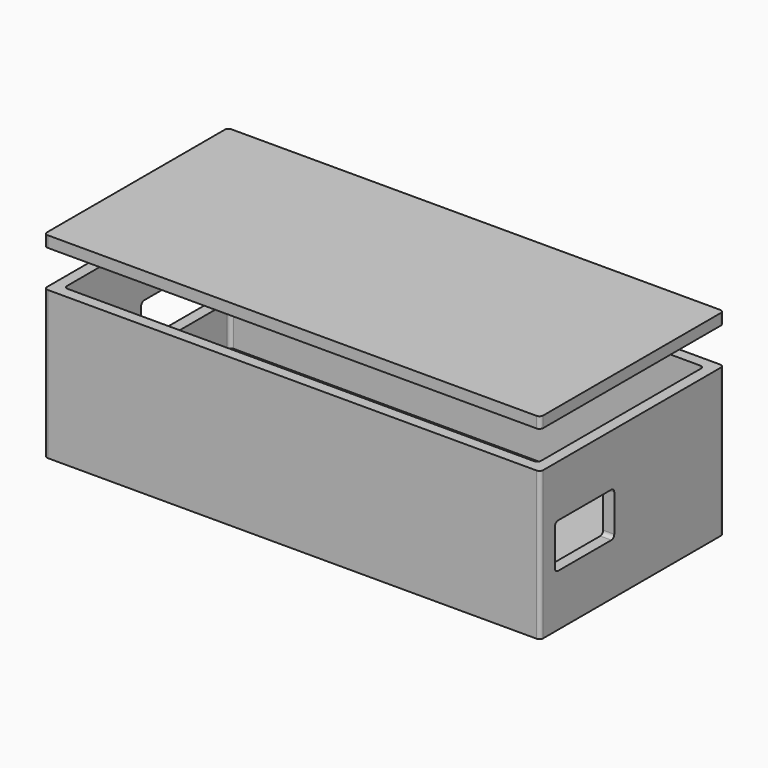
from build123d import *

# Parameters (mm, degrees)
F0_W      = 64
F0_H      = 28
F1_DEPTH  = 1.5
F0_W_2    = 67
F0_H_2    = 31
F2_DEPTH  = 20
F3_W      = 10
F3_H      = 6
F4_DEPTH  = 25
F5_W      = 14
F5_H      = 6
F6_DEPTH  = 25
F7_R      = 0.5
F8_R      = 0.5
F10_W     = 67
F10_H     = 31
F10_W_2   = 64
F10_H_2   = 28
F11_DEPTH = 1.5
F12_DEPTH = 1
F13_R     = 0.5


# Not quite as in the source:
# - a feature names something its author has since deleted; it is built from what else it names


with BuildPart() as f1:
    # F0 (on Top) → F1 (new body)
    with BuildSketch(Plane.XY):
        Rectangle(F0_W, F0_H)
    extrude(amount=F1_DEPTH)

    # F0 (on Top) → F2 (join)
    with BuildSketch(Plane.XY):
        Rectangle(F0_W_2, F0_H_2)
        Rectangle(F0_W, F0_H, mode=Mode.SUBTRACT)
    extrude(amount=F2_DEPTH)

    # F3 (on face) → F4 (cut)
    with BuildSketch(Plane.YZ.offset(33.5)):
        with Locations((-8, 10)):
            Rectangle(F3_W, F3_H)
    extrude(amount=-F4_DEPTH, mode=Mode.SUBTRACT)

    # F5 (on face) → F6 (cut)
    with BuildSketch(Plane(origin=(-33.5, 0, 0), x_dir=(0, -1, 0), z_dir=(-1, 0, 0))):
        with Locations((-6, 10)):
            Rectangle(F5_W, F5_H)
    extrude(amount=-F6_DEPTH, mode=Mode.SUBTRACT)

    # F7
    f7_edges = [f1.edges().sort_by_distance(p)[0] for p in [
        (-32.75, 13, 13),
        (-32.75, 13, 7),
        (-32.75, -1, 13),
        (-32.75, -1, 7),
        (32.75, -13, 13),
        (32.75, -3, 13),
        (32.75, -13, 7),
        (32.75, -3, 7),
    ]]
    fillet(f7_edges, radius=F7_R)

    # F8
    f8_edges = [f1.edges().sort_by_distance(p)[0] for p in [
        (-33.5, -15.5, 10),
        (-33.5, 15.5, 10),
        (33.5, -15.5, 10),
        (33.5, 15.5, 10),
        (32, -14, 10.75),
        (-32, -14, 10.75),
        (-32, 14, 10.75),
        (32, 14, 10.75),
    ]]
    fillet(f8_edges, radius=F8_R)


with BuildPart() as f11:
    # F10 (on offset) → F11 (new body)
    with BuildSketch(Plane.XY.offset(25)):
        Rectangle(F10_W, F10_H)
        Rectangle(F10_W_2, F10_H_2, mode=Mode.SUBTRACT)
        Rectangle(F10_W_2, F10_H_2)
    extrude(amount=F11_DEPTH)

    # F10 (on offset) → F12 (join)
    with BuildSketch(Plane.XY.offset(25)):
        Rectangle(F10_W_2, F10_H_2)
    extrude(amount=-F12_DEPTH)

    # F13
    f13_edges = [f11.edges().sort_by_distance(p)[0] for p in [
        (-32, -14, 24.5),
        (-33.5, -15.5, 25.75),
        (-32, 14, 24.5),
        (-33.5, 15.5, 25.75),
        (32, 14, 24.5),
        (33.5, 15.5, 25.75),
        (32, -14, 24.5),
        (33.5, -15.5, 25.75),
    ]]
    fillet(f13_edges, radius=F13_R)


solid = Compound([f1.part, f11.part])
